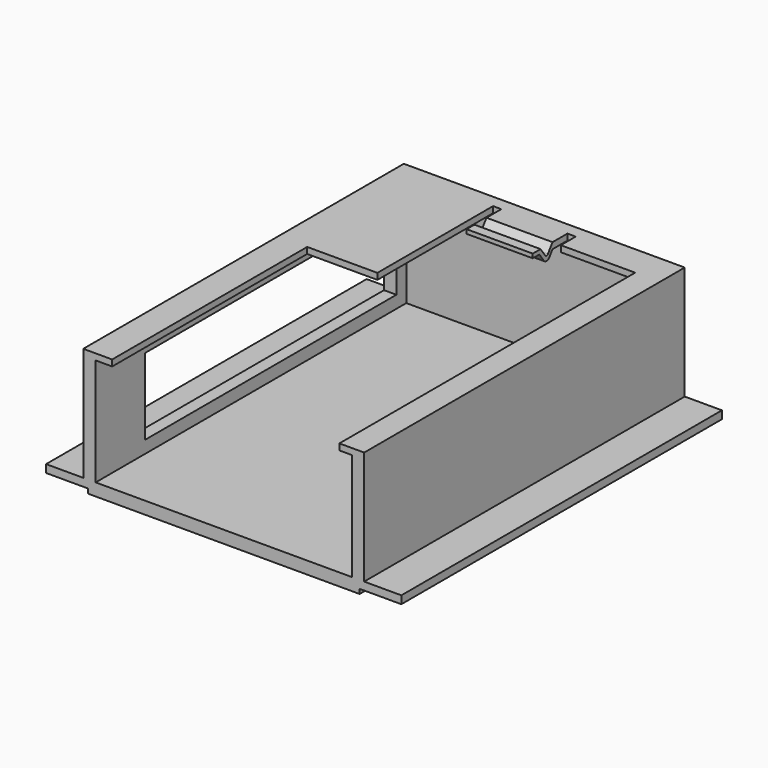
from build123d import *

# Parameters (mm, degrees)
F0_W        = 86
F0_H        = 97
F1_DEPTH    = 3
F2_W        = 68
F2_H        = 97
F3_DEPTH    = 27.5
F4_T        = 3
F4_T3_DEPTH = 103
F7_DEPTH    = 8
F9_DEPTH    = 1.5
F10_W       = 76
F10_H       = 18.5
F11_DEPTH   = 3
F13_DEPTH   = 1.1


# Not quite as in the source:
# - a shell that OpenCascade refuses in one call is made with other operations: the cavity is built on its own and cut out


with BuildPart() as f1:
    # F0 (on Top) → F1 (new body)
    with BuildSketch(Plane.XY):
        with Locations((43, 48.5)):
            Rectangle(F0_W, F0_H)
    extrude(amount=F1_DEPTH)

    # F2 (on face) → F3 (join)
    with BuildSketch(Plane.XY.offset(3)):
        with Locations((43, 48.5)):
            Rectangle(F2_W, F2_H)
    extrude(amount=F3_DEPTH)

    # F4: shell of thickness 3, made by hand


with BuildPart() as f4_core1:
    # F4_t2: copy of F1
    add(f1.part)

    # the walls: a layer under each face that stays
    f4_faces = [f4_core1.faces().sort_by_distance(p)[0] for p in [
        (43, 97, 15.25),
        (86, 48.5, 1.5),
        (0, 48.5, 1.5),
        (43, 48.5, 0),
        (81.5, 48.5, 3),
        (4.5, 48.5, 3),
        (77, 48.5, 16.75),
        (9, 48.5, 16.75),
    ]]
    thicken(f4_faces, amount=-F4_T, mode=Mode.SUBTRACT)

    # F4_s4 → F4_t3 (cut)
    with BuildSketch(Plane.XZ.offset(-100)):
        Polygon((77.03, 3.03), (77, 0), (74, 0), (74, 3), align=None)
        Polygon((8.97, 3.03), (9, 0), (12, 0), (12, 3), align=None)
    extrude(amount=F4_T3_DEPTH, mode=Mode.SUBTRACT)


with BuildPart() as f1_1:
    add(f1.part)

    # what is left inside the walls is the cavity
    f4_cavity = [f4_core1.part.solids().sort_by_distance(p)[0] for p in [
        (43, 31.333333, 3.03),
    ]]
    add(f4_cavity, mode=Mode.SUBTRACT)

    # F6 (on mid) → F7 (join, symmetric)
    with BuildSketch(Plane.YZ.offset(43)):
        with BuildLine():
            Line((94, 29), (94, 30.5))
            Line((94, 30.5), (89.5, 30.5))
            Line((89.5, 30.5), (88.086186224, 28.556006058))
            ThreePointArc((88.086186224, 28.556006058), (87.6818181818, 28.3500919068), (87.2774501397, 28.556006058))
            Line((87.2774501397, 28.556006058), (85.8636363636, 30.5))
            Line((85.8636363636, 30.5), (83.5, 30.5))
            Line((83.5, 30.5), (83.5, 29.5))
            Line((83.5, 29.5), (85.5, 29.5))
            Line((85.5, 29.5), (86.8730820975, 27.6120121159))
            ThreePointArc((86.8730820975, 27.6120121159), (87.6818181818, 27.2001838136), (88.4905542661, 27.6120121159))
            Line((88.4905542661, 27.6120121159), (89.5, 29))
            Line((89.5, 29), (94, 29))
        make_face()
    extrude(amount=F7_DEPTH, both=True)

    # F8 (on face) → F9 (join)
    with BuildSketch(Plane.XY.offset(30.5)):
        Polygon((33, 59), (33, 94), (12, 94), (12, 59), (12, 0), (16, 0), (16, 59), align=None)
        Polygon((59, 94), (53, 94), (53, 89.5), (71, 89.5), (71, 0), (74, 0), (74, 89.5), (74, 94), (71, 94), align=None)
    extrude(amount=-F9_DEPTH)

    # F10 (on face) → F11 (cut, through all)
    with BuildSketch(Plane(origin=(9, 0, 0), x_dir=(0, -1, 0), z_dir=(-1, 0, 0))):
        with Locations((-53, 15.25)):
            Rectangle(F10_W, F10_H)
    extrude(amount=-F11_DEPTH, mode=Mode.SUBTRACT)

    # F12 (on face) → F13 (cut)
    with BuildSketch(Plane(origin=(0, 0, 0), x_dir=(1, 0, 0), z_dir=(0, 0, -1))):
        Polygon((0, 0), (0, -97), (10.1, -97), (75.9, -97), (86, -97), (86, 0), (75.9, 0), (75.9, -93.9), (10.1, -93.9), (10.1, 0), align=None)
    extrude(amount=-F13_DEPTH, mode=Mode.SUBTRACT)


solid = f1_1.part
